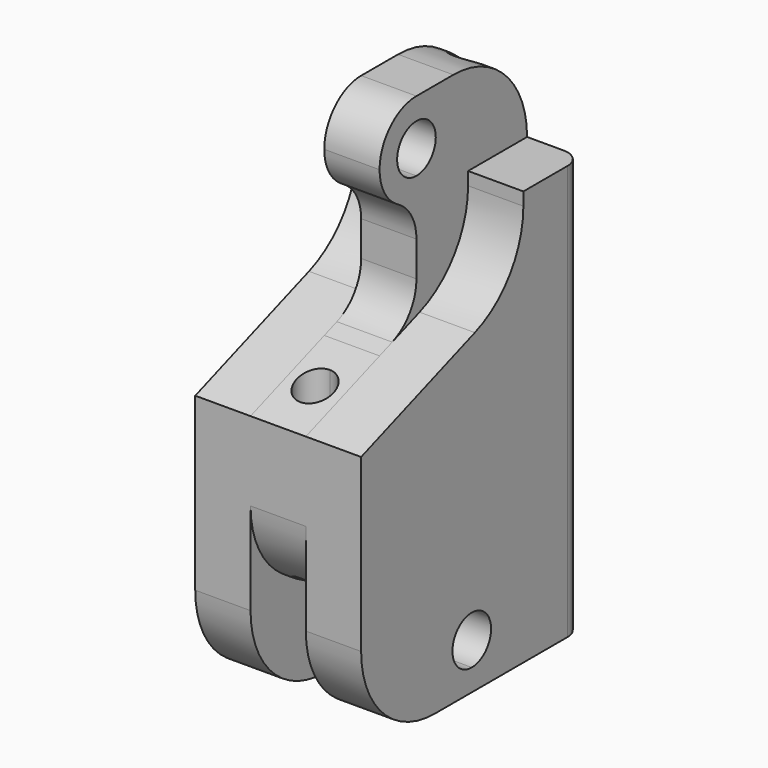
from build123d import *

# Parameters (mm, degrees)
F1_DEPTH     = 15
F3_DEPTH     = 6
F5_DEPTH     = 18
F6_R         = 10
F9_DEPTH     = 6
F10_DEPTH    = 6
F11_R        = 2
F13_DEPTH    = 6
F15_R        = 10
F19_DEPTH    = 50.001
F21_DEPTH    = 45.001
F23_DEPTH    = 6
F24_T1_DEPTH = 6


# Not quite as in the source:
# - a fillet or chamfer that OpenCascade refuses, or shapes differently, is made with other operations: its cross-section is extruded or revolved along the edge and cut away or added


with BuildPart() as f1:
    # F0 (on Front) → F1 (new body, symmetric)
    with BuildSketch(Plane.XZ):
        Polygon((9, -17.5), (9, 17.5), (3, 17.5), (3, 27.5), (-3, 27.5), (-3, 17.5), (-9, 17.5), (-9, -17.5), (-9, -27.5), (-3, -27.5), (-3, -17.5), (3, -17.5), (3, -27.5), (9, -27.5), align=None)
    extrude(amount=F1_DEPTH, both=True)

    # F2 (on face) → F3 (cut)
    with BuildSketch(Plane(origin=(-3, 0, 0), x_dir=(0, -1, 0), z_dir=(-1, 0, 0))):
        with BuildLine():
            ThreePointArc((0, 25.12), (-2.62, 22.5), (0, 19.88))
            Line((0, 19.88), (0, 25.12))
        make_face()
        with BuildLine():
            Line((0, 25.12), (0, 19.88))
            ThreePointArc((0, 19.88), (1.8526197667, 20.6473802333), (2.62, 22.5))
            ThreePointArc((2.62, 22.5), (1.8526197667, 24.3526197667), (0, 25.12))
        make_face()
    extrude(amount=-F3_DEPTH, mode=Mode.SUBTRACT)

    # F4 (on face) → F5 (cut)
    with BuildSketch(Plane(origin=(-9, 0, 0), x_dir=(0, -1, 0), z_dir=(-1, 0, 0))):
        with BuildLine():
            ThreePointArc((0, -25.12), (1.8526197667, -24.3526197667), (2.62, -22.5))
            ThreePointArc((2.62, -22.5), (-1.8526197667, -20.6473802333), (0, -25.12))
        make_face()
    extrude(amount=-F5_DEPTH, mode=Mode.SUBTRACT)

    # F6
    f6_edges = [f1.edges().sort_by_distance(p)[0] for p in [
        (0, 15, 27.5),
        (0, -15, 27.5),
        (6, -15, -27.5),
        (-6, -15, -27.5),
    ]]
    fillet(f6_edges, radius=F6_R)

    # F8 (on face) → F9 (cut)
    with BuildSketch(Plane(origin=(-9, 0, 0), x_dir=(0, -1, 0), z_dir=(-1, 0, 0))):
        with BuildLine():
            ThreePointArc((-7, 16.0872004348), (-5.1915204429, 10.3514360713), (-0.4202014333, 6.690274227))
            Line((-0.4202014333, 6.690274227), (15, 1.0777798989))
            Line((15, 1.0777798989), (15, 17.5))
            Line((15, 17.5), (-7, 17.5))
            Line((-7, 17.5), (-7, 16.0872004348))
        make_face()
    extrude(amount=-F9_DEPTH, mode=Mode.SUBTRACT)

    # F7 (on face) → F10 (cut)
    with BuildSketch(Plane.YZ.offset(9)):
        with BuildLine():
            Line((7, 17.5), (-15, 17.5))
            Line((-15, 17.5), (-15, 1.07778))
            Line((-15, 1.07778), (0.4202014333, 6.6902743281))
            ThreePointArc((0.4202014333, 6.6902743281), (5.1915204429, 10.3514361724), (7, 16.087200536))
            Line((7, 16.087200536), (7, 17.5))
        make_face()
    extrude(amount=-F10_DEPTH, mode=Mode.SUBTRACT)

    # F11
    f11_edges = [f1.edges().sort_by_distance(p)[0] for p in [
        (9, 15, -5),
        (-9, 15, -5),
    ]]
    fillet(f11_edges, radius=F11_R)

    # F12 (on face) → F13 (cut)
    with BuildSketch(Plane(origin=(-3, 0, 0), x_dir=(0, -1, 0), z_dir=(-1, 0, 0))):
        with BuildLine():
            Line((5, 27.5), (0, 27.5))
            ThreePointArc((0, 27.5), (3.5355339059, 26.0355339059), (5, 22.5))
            Line((5, 22.5), (5, 4.7174822415))
            Line((5, 4.7174822415), (15, 1.0777798989))
            Line((15, 1.0777798989), (15, 17.5))
            ThreePointArc((15, 17.5), (12.0710678119, 24.5710678119), (5, 27.5))
        make_face()
    extrude(amount=-F13_DEPTH, mode=Mode.SUBTRACT)

    # F15
    f15_edges = [f1.edges().sort_by_distance(p)[0] for p in [
        (0, -15, -17.5),
    ]]
    fillet(f15_edges, radius=F15_R)

    # F18 (on face) → F19 (cut, through all)
    with BuildSketch(Plane.XY.offset(22.5)):
        with BuildLine():
            ThreePointArc((2, -10), (1.4142135624, -8.5857864376), (0, -8))
            Line((0, -8), (0, -12))
            ThreePointArc((0, -12), (1.4142135624, -11.4142135624), (2, -10))
        make_face()
        with BuildLine():
            Line((0, -12), (0, -8))
            ThreePointArc((0, -8), (-2, -10), (0, -12))
        make_face()
    extrude(amount=-F19_DEPTH, mode=Mode.SUBTRACT)

    # F20 (on face) → F21 (cut, through all)
    with BuildSketch(Plane(origin=(0, 0, -17.5), x_dir=(1, 0, 0), z_dir=(0, 0, -1))):
        with BuildLine():
            ThreePointArc((0, -9), (-2, -11), (0, -13))
            Line((0, -13), (0, -11))
            Line((0, -11), (0, -9))
        make_face()
        with BuildLine():
            Line((0, -11), (0, -13))
            ThreePointArc((0, -13), (1.4142135624, -12.4142135624), (2, -11))
            ThreePointArc((2, -11), (1.4142135624, -9.5857864376), (0, -9))
            Line((0, -9), (0, -11))
        make_face()
    extrude(amount=-F21_DEPTH, mode=Mode.SUBTRACT)

    # F22 (on face) → F23 (cut)
    with BuildSketch(Plane.YZ.offset(3)):
        with BuildLine():
            ThreePointArc((0, 17.5), (-3.5355339059, 18.9644660941), (-5, 22.5))
            Line((-5, 22.5), (-5, 4.7174822415))
            Line((-5, 4.7174822415), (0, 6.5373334129))
            Line((0, 6.5373334129), (0, 17.5))
        make_face()
    extrude(amount=-F23_DEPTH, mode=Mode.SUBTRACT)

    # F24: fillet of radius 5 on 2 edges, made by hand

    # F24_s2 → F24_t1 (join)
    with BuildSketch(Plane.YZ.offset(-3)):
        with BuildLine():
            ThreePointArc((-2.5, 18.1698729811), (-0.6698729811, 16.3397459622), (0, 13.8397459622))
            Line((0, 13.8397459622), (0, 17.5))
            ThreePointArc((0, 17.5), (-1.2940952255, 17.6703708686), (-2.5, 18.1698729811))
        make_face()
        with BuildLine():
            ThreePointArc((-3.2898992834, 5.3399081011), (-0.9042397786, 7.1704890233), (0, 10.038371205))
            Line((0, 10.038371205), (0, 6.5373334129))
            Line((0, 6.5373334129), (-3.2898992834, 5.3399081011))
        make_face()
    extrude(amount=F24_T1_DEPTH)


solid = f1.part
